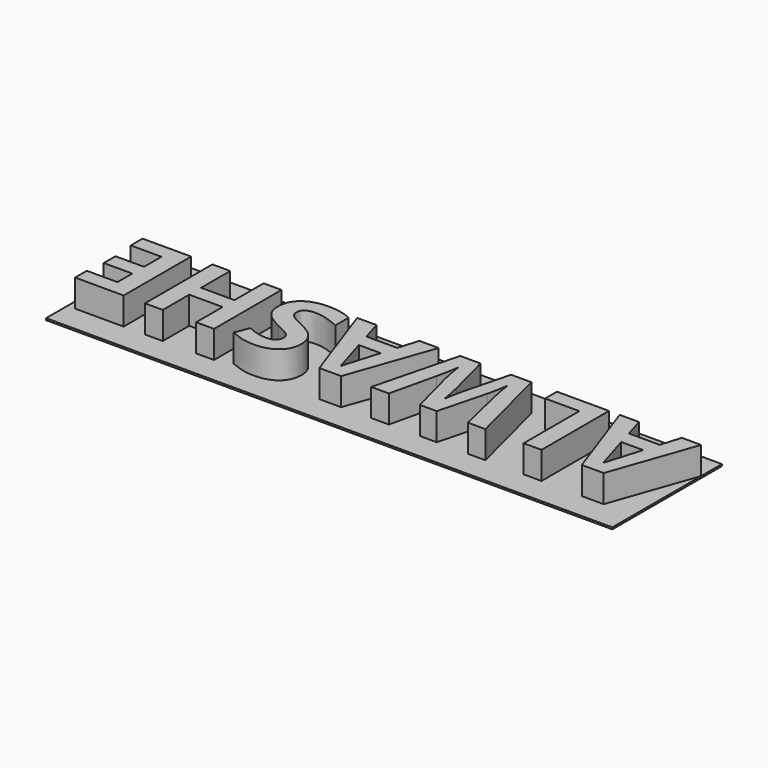
from build123d import *

# Parameters (mm, degrees)
F0_W         = 62
F0_H         = 15
F1_DEPTH     = 0.2
F2_TEXT_SIZE = 12.933928746
F3_DEPTH     = 3


# Not quite as in the source:
# - Text() gives the source's letters only with a copy of the font that has no kerning and outlines rounded to 1/6400 em; it was checked with that copy


with BuildPart() as f1:
    # F0 (on Top) → F1 (new body)
    with BuildSketch(Plane.XY):
        Rectangle(F0_W, F0_H)
    extrude(amount=F1_DEPTH)

    # F2 (on face) → F3 (join)
    with BuildSketch(Plane.XY.offset(0.2)):
        with Locations(Location((31, 4.6562143486), (0, 0, -180))):
            Text('ALWASHE', F2_TEXT_SIZE, font='Open Sans', font_style=FontStyle.BOLD, text_align=(TextAlign.LEFT, TextAlign.BOTTOM))
    extrude(amount=F3_DEPTH)


solid = f1.part
